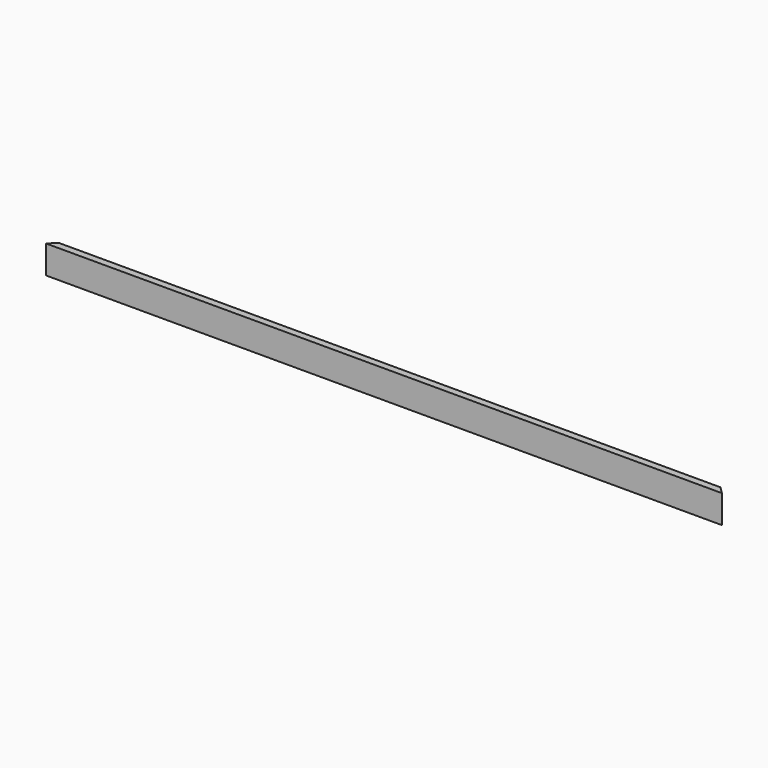
from build123d import *

# Parameters (mm, degrees)
F0_W     = 1828.8
F0_H     = 76.2
F1_DEPTH = 19.05
F2_SIZE  = 19.04999


# Not quite as in the source:
# - a fillet or chamfer is up to 0.001 mm smaller than in the source, because OpenCascade refuses the exact size


with BuildPart() as f1:
    # F0 (on Front) → F1 (new body)
    with BuildSketch(Plane.XZ):
        Rectangle(F0_W, F0_H)
    extrude(amount=F1_DEPTH)

    # F2 (size 19.05 in the source; OpenCascade refuses exactly that, so slightly less here)
    f2_edges = [f1.edges().sort_by_distance(p)[0] for p in [
        (-914.4, 0, 0),
        (914.4, 0, 0),
    ]]
    chamfer(f2_edges, length=F2_SIZE)


solid = f1.part
